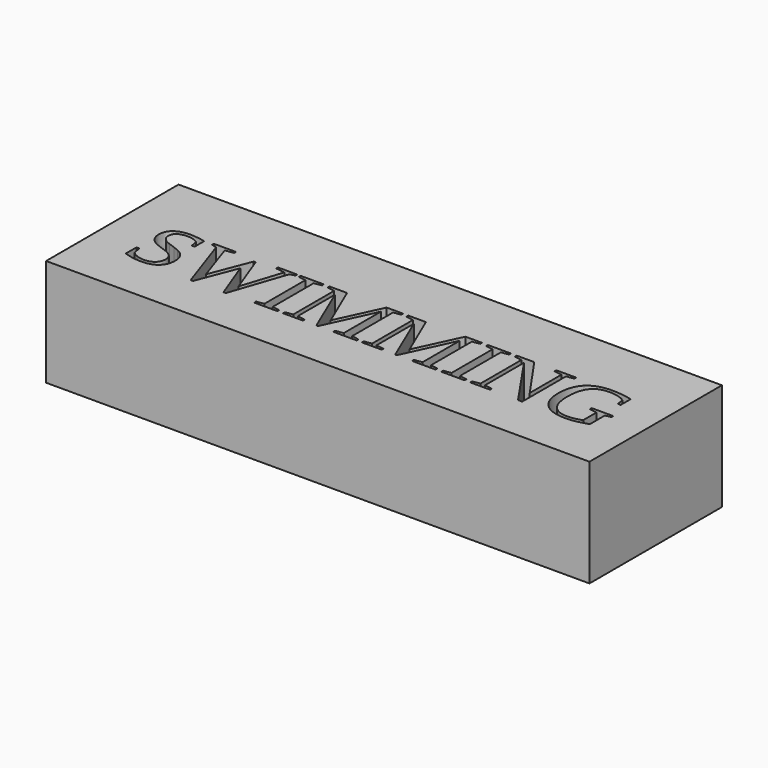
from build123d import *

# Parameters (mm, degrees)
F0_W     = 193.128593266
F0_H     = 58.8438659906
F1_DEPTH = 38.1


with BuildPart() as f1:
    # F0 (on Top) → F1 (new body)
    with BuildSketch(Plane.XY):
        with Locations((6.6010765731, -9.8073109984)):
            Rectangle(F0_W, F0_H)
        with BuildLine():
            Line((-75.4900585158, -21.9018592134), (-75.4900585158, -17.1315958783))
            Line((-75.4900585158, -17.1315958783), (-74.4857925505, -17.1315958783))
            Line((-74.4857925505, -17.1315958783), (-73.9491994612, -19.9130187723))
            add(Edge.make_bspline(
                [(-73.9491994612, -19.9130187723), (-73.3781462652, -20.636681012), (-71.9874348182, -21.1905041547)],
                knots=[0, 0, 0, 1, 1, 1], degree=2))
            add(Edge.make_bspline(
                [(-71.9874348182, -21.1905041547), (-70.5967233712, -21.7443272973), (-69.242933467, -21.7443272973)],
                knots=[0, 0, 0, 1, 1, 1], degree=2))
            add(Edge.make_bspline(
                [(-69.242933467, -21.7443272973), (-67.0867153651, -21.7443272973), (-65.8806116323, -20.6440653206)],
                knots=[0, 0, 0, 1, 1, 1], degree=2))
            add(Edge.make_bspline(
                [(-65.8806116323, -20.6440653206), (-64.6745078995, -19.5438033439), (-64.6745078995, -17.6091144991)],
                knots=[0, 0, 0, 1, 1, 1], degree=2))
            add(Edge.make_bspline(
                [(-64.6745078995, -17.6091144991), (-64.6745078995, -16.5014682138), (-65.1421807755, -15.7778059741)],
                knots=[0, 0, 0, 1, 1, 1], degree=2))
            add(Edge.make_bspline(
                [(-65.1421807755, -15.7778059741), (-65.6098536515, -15.0541437344), (-66.3728988702, -14.554472188)],
                knots=[0, 0, 0, 1, 1, 1], degree=2))
            add(Edge.make_bspline(
                [(-66.3728988702, -14.554472188), (-67.1359440889, -14.0548006415), (-68.1032885113, -13.7077381388)],
                knots=[0, 0, 0, 1, 1, 1], degree=2))
            add(Edge.make_bspline(
                [(-68.1032885113, -13.7077381388), (-69.0706329338, -13.3606756361), (-70.0945903886, -13.0062288249)],
                knots=[0, 0, 0, 1, 1, 1], degree=2))
            add(Edge.make_bspline(
                [(-70.0945903886, -13.0062288249), (-71.1185478434, -12.6517820136), (-72.088353702, -12.2210306804)],
                knots=[0, 0, 0, 1, 1, 1], degree=2))
            add(Edge.make_bspline(
                [(-72.088353702, -12.2210306804), (-73.0581595606, -11.7902793473), (-73.8187433432, -11.1306144485)],
                knots=[0, 0, 0, 1, 1, 1], degree=2))
            add(Edge.make_bspline(
                [(-73.8187433432, -11.1306144485), (-74.5793271257, -10.4709495498), (-75.0494614379, -9.4937593826)],
                knots=[0, 0, 0, 1, 1, 1], degree=2))
            add(Edge.make_bspline(
                [(-75.0494614379, -9.4937593826), (-75.51959575, -8.5165692154), (-75.51959575, -7.0840133531)],
                knots=[0, 0, 0, 1, 1, 1], degree=2))
            add(Edge.make_bspline(
                [(-75.51959575, -7.0840133531), (-75.51959575, -4.6225771637), (-73.673518608, -3.2220199719)],
                knots=[0, 0, 0, 1, 1, 1], degree=2))
            add(Edge.make_bspline(
                [(-73.673518608, -3.2220199719), (-71.8274414659, -1.8214627802), (-68.5488084616, -1.8214627802)],
                knots=[0, 0, 0, 1, 1, 1], degree=2))
            add(Edge.make_bspline(
                [(-68.5488084616, -1.8214627802), (-66.0578350379, -1.8214627802), (-63.1336488449, -2.4860505513)],
                knots=[0, 0, 0, 1, 1, 1], degree=2))
            Line((-63.1336488449, -2.4860505513), (-63.1336488449, -6.7787952656))
            Line((-63.1336488449, -6.7787952656), (-64.1329919378, -6.7787952656))
            Line((-64.1329919378, -6.7787952656), (-64.6745078995, -4.2533617353))
            add(Edge.make_bspline(
                [(-64.6745078995, -4.2533617353), (-66.2399813159, -3.1161782158), (-68.5488084616, -3.1161782158)],
                knots=[0, 0, 0, 1, 1, 1], degree=2))
            add(Edge.make_bspline(
                [(-68.5488084616, -3.1161782158), (-70.6114919883, -3.1161782158), (-71.7732898697, -3.9555279564)],
                knots=[0, 0, 0, 1, 1, 1], degree=2))
            add(Edge.make_bspline(
                [(-71.7732898697, -3.9555279564), (-72.9350877512, -4.794877697), (-72.9350877512, -6.2717394106)],
                knots=[0, 0, 0, 1, 1, 1], degree=2))
            add(Edge.make_bspline(
                [(-72.9350877512, -6.2717394106), (-72.9350877512, -7.2710825035), (-72.464953439, -7.9307474023)],
                knots=[0, 0, 0, 1, 1, 1], degree=2))
            add(Edge.make_bspline(
                [(-72.464953439, -7.9307474023), (-71.9948191268, -8.590412301), (-71.2342353443, -9.0605466132)],
                knots=[0, 0, 0, 1, 1, 1], degree=2))
            add(Edge.make_bspline(
                [(-71.2342353443, -9.0605466132), (-70.4736515617, -9.5306809254), (-69.4964613945, -9.8703591195)],
                knots=[0, 0, 0, 1, 1, 1], degree=2))
            add(Edge.make_bspline(
                [(-69.4964613945, -9.8703591195), (-68.5192712273, -10.2100373137), (-67.4953137726, -10.5694069973)],
                knots=[0, 0, 0, 1, 1, 1], degree=2))
            add(Edge.make_bspline(
                [(-67.4953137726, -10.5694069973), (-66.4713563178, -10.928776681), (-65.4941661506, -11.384142376)],
                knots=[0, 0, 0, 1, 1, 1], degree=2))
            add(Edge.make_bspline(
                [(-65.4941661506, -11.384142376), (-64.5169759834, -11.8395080711), (-63.7563922008, -12.5385559489)],
                knots=[0, 0, 0, 1, 1, 1], degree=2))
            add(Edge.make_bspline(
                [(-63.7563922008, -12.5385559489), (-62.9958084183, -13.2376038267), (-62.5256741061, -14.2467926643)],
                knots=[0, 0, 0, 1, 1, 1], degree=2))
            add(Edge.make_bspline(
                [(-62.5256741061, -14.2467926643), (-62.0555397939, -15.255981502), (-62.0555397939, -16.7328432156)],
                knots=[0, 0, 0, 1, 1, 1], degree=2))
            add(Edge.make_bspline(
                [(-62.0555397939, -16.7328432156), (-62.0555397939, -19.7161038772), (-63.8868483189, -21.3554203793)],
                knots=[0, 0, 0, 1, 1, 1], degree=2))
            add(Edge.make_bspline(
                [(-63.8868483189, -21.3554203793), (-65.7181568438, -22.9947368815), (-69.164167509, -22.9947368815)],
                knots=[0, 0, 0, 1, 1, 1], degree=2))
            add(Edge.make_bspline(
                [(-69.164167509, -22.9947368815), (-70.828098373, -22.9947368815), (-72.504336418, -22.701825975)],
                knots=[0, 0, 0, 1, 1, 1], degree=2))
            add(Edge.make_bspline(
                [(-72.504336418, -22.701825975), (-74.180574463, -22.4089150684), (-75.4900585158, -21.9018592134)],
                knots=[0, 0, 0, 1, 1, 1], degree=2))
        make_face(mode=Mode.SUBTRACT)
        Polygon((-32.2278560506, -3.2687872595), (-38.9672683373, -23.1621145424), (-39.7844651521, -23.1621145424), (-45.1356274279, -8.9448591123), (-50.6295530027, -23.1621145424), (-51.4467498176, -23.1621145424), (-58.274773807, -3.2687872595), (-60.0765450977, -2.8700345969), (-60.0765450977, -2.052837782), (-52.1999492915, -2.052837782), (-52.1999492915, -2.8700345969), (-55.2275158045, -3.2687872595), (-50.3194120428, -17.8060293942), (-44.7664119995, -3.5001622613), (-44.0772098665, -3.5001622613), (-38.7211247183, -17.8060293942), (-34.0443959584, -3.2687872595), (-37.2590316218, -2.8700345969), (-37.2590316218, -2.052837782), (-30.4310076324, -2.052837782), (-30.4310076324, -2.8700345969), align=None, mode=Mode.SUBTRACT)
        Polygon((-23.6275980048, -3.2687872595), (-23.6275980048, -21.4538778269), (-20.9840155374, -21.8673991067), (-20.9840155374, -22.6845959216), (-29.2298267719, -22.6845959216), (-29.2298267719, -21.8673991067), (-26.5813214321, -21.4538778269), (-26.5813214321, -3.2687872595), (-29.2298267719, -2.8700345969), (-29.2298267719, -2.052837782), (-20.9840155374, -2.052837782), (-20.9840155374, -2.8700345969), align=None, mode=Mode.SUBTRACT)
        Polygon((1.6168915538, -4.9474867407), (-6.6141510636, -22.6845959216), (-7.1556670253, -22.6845959216), (-14.7073532544, -4.9474867407), (-14.7073532544, -21.4538778269), (-11.9357761051, -21.8673991067), (-11.9357761051, -22.6845959216), (-18.9705607345, -22.6845959216), (-18.9705607345, -21.8673991067), (-16.3220553947, -21.4538778269), (-16.3220553947, -3.2687872595), (-18.9705607345, -2.8700345969), (-18.9705607345, -2.052837782), (-12.7234356857, -2.052837782), (-6.0135606334, -17.7469549257), (1.3067505939, -2.052837782), (7.2141974485, -2.052837782), (7.2141974485, -2.8700345969), (4.5706149811, -3.2687872595), (4.5706149811, -21.4538778269), (7.2141974485, -21.8673991067), (7.2141974485, -22.6845959216), (-1.1546855955, -22.6845959216), (-1.1546855955, -21.8673991067), (1.6168915538, -21.4538778269), align=None, mode=Mode.SUBTRACT)
        Polygon((29.6329582617, -4.9474867407), (21.4019156443, -22.6845959216), (20.8603996826, -22.6845959216), (13.3087134535, -4.9474867407), (13.3087134535, -21.4538778269), (16.0802906028, -21.8673991067), (16.0802906028, -22.6845959216), (9.0455059734, -22.6845959216), (9.0455059734, -21.8673991067), (11.6940113132, -21.4538778269), (11.6940113132, -3.2687872595), (9.0455059734, -2.8700345969), (9.0455059734, -2.052837782), (15.2926310222, -2.052837782), (22.0025060745, -17.7469549257), (29.3228173018, -2.052837782), (35.2302641564, -2.052837782), (35.2302641564, -2.8700345969), (32.586681689, -3.2687872595), (32.586681689, -21.4538778269), (35.2302641564, -21.8673991067), (35.2302641564, -22.6845959216), (26.8613811124, -22.6845959216), (26.8613811124, -21.8673991067), (29.6329582617, -21.4538778269), align=None, mode=Mode.SUBTRACT)
        Polygon((42.8951764502, -3.2687872595), (42.8951764502, -21.4538778269), (45.5387589177, -21.8673991067), (45.5387589177, -22.6845959216), (37.2929476831, -22.6845959216), (37.2929476831, -21.8673991067), (39.9414530229, -21.4538778269), (39.9414530229, -3.2687872595), (37.2929476831, -2.8700345969), (37.2929476831, -2.052837782), (45.5387589177, -2.052837782), (45.5387589177, -2.8700345969), align=None, mode=Mode.SUBTRACT)
        Polygon((64.4130516181, -17.3285107735), (64.4130516181, -3.2687872595), (61.6463973412, -2.8700345969), (61.6463973412, -2.052837782), (68.6762590981, -2.052837782), (68.6762590981, -2.8700345969), (66.0326766307, -3.2687872595), (66.0326766307, -22.6845959216), (64.5361234275, -22.6845959216), (51.8154212007, -4.1302899258), (51.8154212007, -21.4538778269), (54.5869983499, -21.8673991067), (54.5869983499, -22.6845959216), (47.5522137206, -22.6845959216), (47.5522137206, -21.8673991067), (50.2007190604, -21.4538778269), (50.2007190604, -3.2687872595), (47.5522137206, -2.8700345969), (47.5522137206, -2.052837782), (53.7993387693, -2.052837782), align=None, mode=Mode.SUBTRACT)
        with BuildLine():
            Line((89.155408194, -14.9015346907), (89.155408194, -21.6064868707))
            add(Edge.make_bspline(
                [(89.155408194, -21.6064868707), (87.3684055205, -22.1923086837), (85.4460238566, -22.5935227826)],
                knots=[0, 0, 0, 1, 1, 1], degree=2))
            add(Edge.make_bspline(
                [(85.4460238566, -22.5935227826), (83.5236421927, -22.9947368815), (81.3083496222, -22.9947368815)],
                knots=[0, 0, 0, 1, 1, 1], degree=2))
            add(Edge.make_bspline(
                [(81.3083496222, -22.9947368815), (76.2919426682, -22.9947368815), (73.4932897208, -20.2846956369)],
                knots=[0, 0, 0, 1, 1, 1], degree=2))
            add(Edge.make_bspline(
                [(73.4932897208, -20.2846956369), (70.6946367735, -17.5746543924), (70.6946367735, -12.6074761622)],
                knots=[0, 0, 0, 1, 1, 1], degree=2))
            add(Edge.make_bspline(
                [(70.6946367735, -12.6074761622), (70.6946367735, -7.1923165455), (73.4096008904, -4.5068896628)],
                knots=[0, 0, 0, 1, 1, 1], degree=2))
            add(Edge.make_bspline(
                [(73.4096008904, -4.5068896628), (76.1245650073, -1.8214627802), (81.3674240907, -1.8214627802)],
                knots=[0, 0, 0, 1, 1, 1], degree=2))
            add(Edge.make_bspline(
                [(81.3674240907, -1.8214627802), (85.1235757158, -1.8214627802), (88.6138922324, -2.7469627874)],
                knots=[0, 0, 0, 1, 1, 1], degree=2))
            Line((88.6138922324, -2.7469627874), (88.6138922324, -7.1775479283))
            Line((88.6138922324, -7.1775479283), (87.5850119052, -7.1775479283))
            Line((87.5850119052, -7.1775479283), (87.166567753, -4.6225771637))
            add(Edge.make_bspline(
                [(87.166567753, -4.6225771637), (86.1081501916, -3.8693776898), (84.6239041693, -3.4607792823)],
                knots=[0, 0, 0, 1, 1, 1], degree=2))
            add(Edge.make_bspline(
                [(84.6239041693, -3.4607792823), (83.1396581471, -3.0521808749), (81.4904959002, -3.0521808749)],
                knots=[0, 0, 0, 1, 1, 1], degree=2))
            add(Edge.make_bspline(
                [(81.4904959002, -3.0521808749), (77.5521979972, -3.0521808749), (75.730735217, -5.4003909996)],
                knots=[0, 0, 0, 1, 1, 1], degree=2))
            add(Edge.make_bspline(
                [(75.730735217, -5.4003909996), (73.9092724368, -7.7486011243), (73.9092724368, -12.5779389279)],
                knots=[0, 0, 0, 1, 1, 1], degree=2))
            add(Edge.make_bspline(
                [(73.9092724368, -12.5779389279), (73.9092724368, -17.1168272612), (75.7848868132, -19.4625759497)],
                knots=[0, 0, 0, 1, 1, 1], degree=2))
            add(Edge.make_bspline(
                [(75.7848868132, -19.4625759497), (77.6605011895, -21.8083246382), (81.3378868565, -21.8083246382)],
                knots=[0, 0, 0, 1, 1, 1], degree=2))
            add(Edge.make_bspline(
                [(81.3378868565, -21.8083246382), (82.6326022921, -21.8083246382), (84.047928101, -21.5006451145)],
                knots=[0, 0, 0, 1, 1, 1], degree=2))
            add(Edge.make_bspline(
                [(84.047928101, -21.5006451145), (85.4632539099, -21.1929655908), (86.2016847668, -20.7597528215)],
                knots=[0, 0, 0, 1, 1, 1], degree=2))
            Line((86.2016847668, -20.7597528215), (86.2016847668, -14.9015346907))
            Line((86.2016847668, -14.9015346907), (83.5531794269, -14.4978591556))
            Line((83.5531794269, -14.4978591556), (83.5531794269, -13.670816596))
            Line((83.5531794269, -13.670816596), (91.168862997, -13.670816596))
            Line((91.168862997, -13.670816596), (91.168862997, -14.4978591556))
            Line((91.168862997, -14.4978591556), (89.155408194, -14.9015346907))
        make_face(mode=Mode.SUBTRACT)
    extrude(amount=F1_DEPTH)


solid = f1.part
